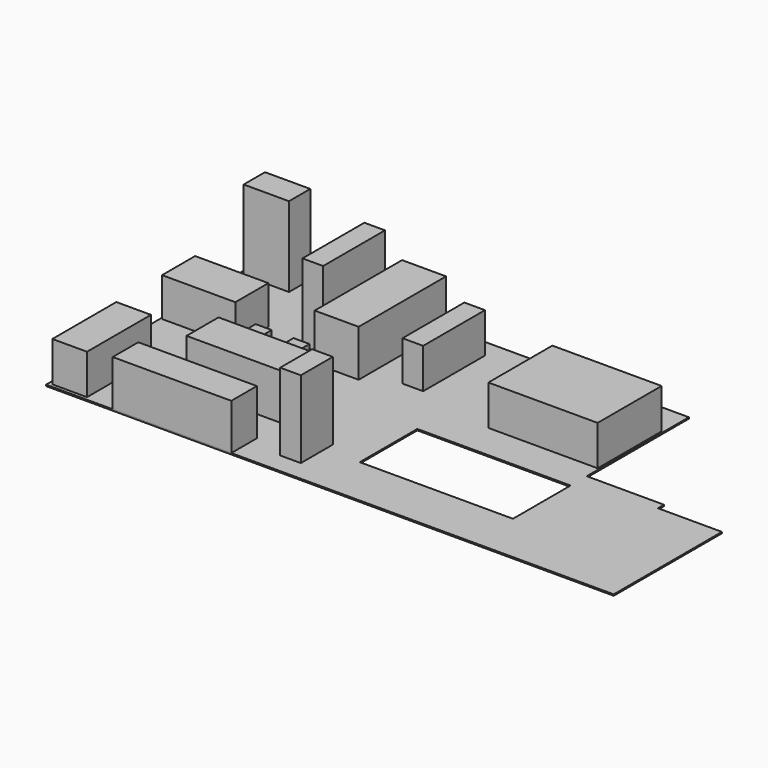
from build123d import *

# Parameters (mm, degrees)
F2_DEPTH  = 901.7
F0_W      = 2260.6
F0_H      = 609.6
F0_W_2    = 609.6
F0_H_2    = 2438.4
F4_DEPTH  = 25.4
F7_W      = 838.2
F7_H      = 2082.8
F8_DEPTH  = 889
F9_W      = 393.7
F9_H      = 1473.2
F10_DEPTH = 762
F11_W     = 863.6
F11_H     = 508
F12_DEPTH = 1524
F13_W     = 1397
F13_H     = 787.4
F14_DEPTH = 736.6
F15_W     = 393.7
F15_H     = 762
F16_DEPTH = 1473.2
F17_W     = 393.7
F17_H     = 1473.2
F18_DEPTH = 1473.2
F19_W     = 304.8
F19_H     = 304.8
F20_DEPTH = 736.6
F21_W     = 660.4
F21_H     = 1524
F22_DEPTH = 762
F23_W     = 2082.8
F23_H     = 1524
F24_DEPTH = 762


# Not quite as in the source:
# - the program builds the solid bodies; features that only make, move or delete a surface that nothing else refers to are left out


with BuildPart() as f2:
    # F0 (on Top) → F2 (new body)
    with BuildSketch(Plane.XY):
        Polygon((-1270, -1358.9), (-1270, -952.5), (-1270, -596.9), (-3098.8, -596.9), (-3098.8, -1358.9), align=None)
    extrude(amount=F2_DEPTH)


with BuildPart() as f2b:
    # F0 (on Top) → F2, piece 2 (new body)
    with BuildSketch(Plane.XY):
        with Locations((-2400.3, -2273.3)):
            Rectangle(F0_W, F0_H)
    extrude(amount=F2_DEPTH)


with BuildPart() as f4:
    # F0 (on Top) → F4 (new body)
    with BuildSketch(Plane.XY):
        Polygon((-812.8, -2578.1), (4800.6, -2578.1), (4800.6, -1612.9), (3327.4, -1612.9), (406.4, -1612.9), (406.4, -241.3), (406.4, 139.7), (-203.2, 139.7), (-203.2, 2578.1), (-4800.6, 2578.1), (-4800.6, -2578.1), (-3530.6, -2578.1), (-3530.6, -1968.5), (-1270, -1968.5), (-1270, -1358.9), (-3098.8, -1358.9), (-3098.8, -596.9), (-1270, -596.9), (-1270, -952.5), (-812.8, -952.5), align=None)
        Polygon((4800.6, -1612.9), (4800.6, -2578.1), (6019.8, -2578.1), (6019.8, 0), (4800.6, 0), align=None)
        Polygon((-1270, -2578.1), (-812.8, -2578.1), (-812.8, -952.5), (-1270, -952.5), (-1270, -1358.9), (-1270, -1968.5), align=None)
        Polygon((3327.4, -1612.9), (4800.6, -1612.9), (4800.6, 0), (4800.6, 144.5753626943), (3327.4, 144.5753626943), (3327.4, -241.3), align=None)
        with Locations((-2400.3, -2273.3)):
            Rectangle(F0_W, F0_H)
        Polygon((406.4, -241.3), (3327.4, -241.3), (3327.4, 144.5753626943), (3327.4, 2578.1), (406.4, 2578.1), (406.4, 139.7), align=None)
        with Locations((101.6, 1358.9)):
            Rectangle(F0_W_2, F0_H_2)
    extrude(amount=F4_DEPTH)


with BuildPart() as f8:
    # F7 (on face) → F8 (new body)
    with BuildSketch(Plane.XY.offset(25.4)):
        with Locations((-1684.229016304, 1491.4646148682)):
            Rectangle(F7_W, F7_H)
    extrude(amount=F8_DEPTH)


with BuildPart() as f10:
    # F9 (on face) → F10 (new body)
    with BuildSketch(Plane.XY.offset(25.4)):
        with Locations((-481.2808632851, 1498.0827569962)):
            Rectangle(F9_W, F9_H)
    extrude(amount=F10_DEPTH)


with BuildPart() as f12:
    # F11 (on face) → F12 (new body)
    with BuildSketch(Plane.XY.offset(25.4)):
        with Locations((-4273.6654281616, 2264.9219036102)):
            Rectangle(F11_W, F11_H)
    extrude(amount=F12_DEPTH)


with BuildPart() as f14:
    # F13 (on face) → F14 (new body)
    with BuildSketch(Plane.XY.offset(25.4)):
        with Locations((-4075.2243995667, 545.2215075493)):
            Rectangle(F13_W, F13_H)
    extrude(amount=F14_DEPTH)


with BuildPart() as f16:
    # F15 (on face) → F16 (new body)
    with BuildSketch(Plane.XY.offset(25.4)):
        with Locations((-456.366866827, -1803.3801317215)):
            Rectangle(F15_W, F15_H)
    extrude(amount=F16_DEPTH)


with BuildPart() as f18:
    # F17 (on face) → F18 (new body)
    with BuildSketch(Plane.XY.offset(25.4)):
        with Locations((-2397.4113569062, 1510.4005336761)):
            Rectangle(F17_W, F17_H)
    extrude(amount=F18_DEPTH)


with BuildPart() as f20:
    # F19 (on face) → F20 (new body)
    with BuildSketch(Plane.XY.offset(25.4)):
        with Locations((-1825.1785008743, -363.2096648216)):
            Rectangle(F19_W, F19_H)
    extrude(amount=F20_DEPTH)


with BuildPart() as f20b:
    # F19 (on face) → F20, piece 2 (new body)
    with BuildSketch(Plane.XY.offset(25.4)):
        with Locations((-2546.5385913849, -363.2096648216)):
            Rectangle(F19_W, F19_H)
    extrude(amount=F20_DEPTH)


with BuildPart() as f22:
    # F21 (on face) → F22 (new body)
    with BuildSketch(Plane.XY.offset(25.4)):
        with Locations((-4402.7910232544, -1750.9953975677)):
            Rectangle(F21_W, F21_H)
    extrude(amount=F22_DEPTH)


with BuildPart() as f24:
    # F23 (on face) → F24 (new body)
    with BuildSketch(Plane.XY.offset(25.4)):
        with Locations((2253.6647319794, 1206.5)):
            Rectangle(F23_W, F23_H)
    extrude(amount=F24_DEPTH)


solid = Compound([f2.part, f2b.part, f4.part, f8.part, f10.part, f12.part, f14.part, f16.part, f18.part, f20.part, f20b.part, f22.part, f24.part])
